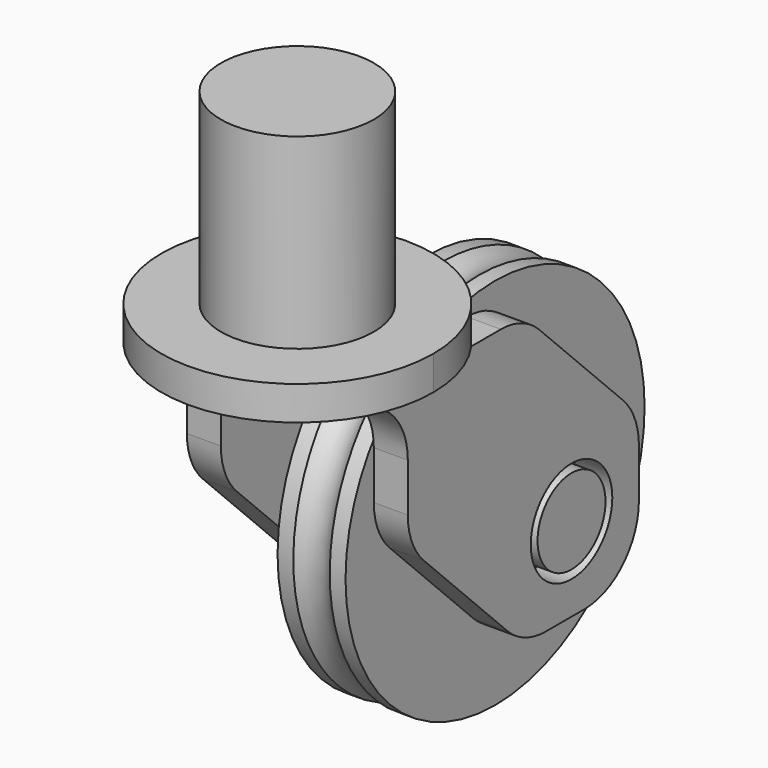
from build123d import *

# Parameters (mm, degrees)
F1_DEPTH  = 13
F2_DEPTH  = 2
F3_DEPTH  = 17
F5_DEPTH  = 14
F6_R      = 4
F7_D      = 6
F8_R      = 11
F8_R_2    = 4.05
F9_DEPTH  = 2
F8_R_3    = 2.5
F10_DEPTH = 6.5
F8_R_4    = 4
F11_DEPTH = 4
F13_R     = 1.5


with BuildPart() as f1:
    # F0 (on Top) → F1 (new body)
    with BuildSketch(Plane.XY):
        with BuildLine():
            ThreePointArc((-4.5, 0), (0, -4.5), (4.5, 0))
            ThreePointArc((4.5, 0), (0, 4.5), (-4.5, 0))
        make_face()
    extrude(amount=F1_DEPTH)

    # F0 (on Top) → F2 (join)
    with BuildSketch(Plane.XY):
        with BuildLine():
            ThreePointArc((-4.5, 0), (0, 4.5), (4.5, 0))
            Line((4.5, 0), (4.5, 6.6143782777))
            ThreePointArc((4.5, 6.6143782777), (0, 8), (-4.5, 6.6143782777))
            Line((-4.5, 6.6143782777), (-4.5, 0))
        make_face()
        with BuildLine():
            Line((-6.5, 0), (-4.5, 0))
            Line((-4.5, 0), (-4.5, 6.6143782777))
            ThreePointArc((-4.5, 6.6143782777), (-5.5858120852, 5.7270152217), (-6.5, 4.6636895265))
            Line((-6.5, 4.6636895265), (-6.5, 0))
        make_face()
        with BuildLine():
            Line((6.5, 0), (4.5, 0))
            ThreePointArc((4.5, 0), (0, -4.5), (-4.5, 0))
            Line((-4.5, 0), (-6.5, 0))
            Line((-6.5, 0), (-6.5, 4.6636895265))
            ThreePointArc((-6.5, 4.6636895265), (-2.4494897428, -7.6157731059), (8, 0))
            ThreePointArc((8, 0), (7.6157731059, 2.4494897428), (6.5, 4.6636895265))
            Line((6.5, 4.6636895265), (6.5, 0))
        make_face()
        with BuildLine():
            Line((4.5, 6.6143782777), (4.5, 0))
            Line((4.5, 0), (6.5, 0))
            Line((6.5, 0), (6.5, 4.6636895265))
            ThreePointArc((6.5, 4.6636895265), (5.5858120852, 5.7270152217), (4.5, 6.6143782777))
        make_face()
    extrude(amount=F2_DEPTH)

    # F0 (on Top) → F3 (join)
    with BuildSketch(Plane.XY):
        with BuildLine():
            ThreePointArc((-6.5, 4.6636895265), (-5.5858120852, 5.7270152217), (-4.5, 6.6143782777))
            Line((-4.5, 6.6143782777), (-4.5, 17))
            Line((-4.5, 17), (-6.5, 17))
            Line((-6.5, 17), (-6.5, 4.6636895265))
        make_face()
        with BuildLine():
            Line((4.5, 17), (4.5, 6.6143782777))
            ThreePointArc((4.5, 6.6143782777), (5.5858120852, 5.7270152217), (6.5, 4.6636895265))
            Line((6.5, 4.6636895265), (6.5, 17))
            Line((6.5, 17), (4.5, 17))
        make_face()
        with BuildLine():
            Line((-6.5, 0), (-4.5, 0))
            Line((-4.5, 0), (-4.5, 6.6143782777))
            ThreePointArc((-4.5, 6.6143782777), (-5.5858120852, 5.7270152217), (-6.5, 4.6636895265))
            Line((-6.5, 4.6636895265), (-6.5, 0))
        make_face()
        with BuildLine():
            Line((4.5, 6.6143782777), (4.5, 0))
            Line((4.5, 0), (6.5, 0))
            Line((6.5, 0), (6.5, 4.6636895265))
            ThreePointArc((6.5, 4.6636895265), (5.5858120852, 5.7270152217), (4.5, 6.6143782777))
        make_face()
    extrude(amount=-F3_DEPTH)

    # F4 (on face) → F5 (cut)
    with BuildSketch(Plane(origin=(-6.5, 0, 0), x_dir=(0, -1, 0), z_dir=(-1, 0, 0))):
        Polygon((-17, 0), (-17, -8.5), (-8.5, 0), align=None)
        Polygon((0, -17), (0, -8.5), (-8.5, -17), align=None)
    extrude(amount=-F5_DEPTH, mode=Mode.SUBTRACT)

    # F6
    f6_edges = [f1.edges().sort_by_distance(p)[0] for p in [
        (-5.5, 17, -17),
        (5.5, 17, -17),
        (-5.5, 0, 0),
        (5.5, 0, 0),
        (-5.5, 0, -8.5),
        (5.5, 0, -8.5),
        (5.5, 8.5, -17),
        (-5.5, 8.5, -17),
        (5.5, 17, -8.5),
        (-5.5, 17, -8.5),
        (5.5, 8.5, 0),
        (-5.5, 8.5, 0),
    ]]
    fillet(f6_edges, radius=F6_R)

    # F7 (through all)
    with Locations(Plane(origin=(-6.5, 0, 0), x_dir=(0, -1, 0), z_dir=(-1, 0, 0))):
        with Locations((-12.0428986898, -12.0576173155)):
            Hole(F7_D / 2)


with BuildPart() as f9:
    # F8 (on Right) → F9 (new body, symmetric)
    with BuildSketch(Plane.YZ):
        with Locations((12.0428986898, -12.0576173155)):
            Circle(F8_R)
        with Locations((12.0428986898, -12.0576173155)):
            Circle(F8_R_2, mode=Mode.SUBTRACT)
    extrude(amount=F9_DEPTH, both=True)

    # F13 (on offset) → F14 (revolve, cut)
    with BuildSketch(Plane.XZ.offset(-11)):
        with Locations((0, -24.0576173155)):
            Circle(F13_R)
    revolve(axis=Axis((2, 12.0428986898, -12.0576173155), (1, 0, 0)), mode=Mode.SUBTRACT)


with BuildPart() as f10:
    # F8 (on Right) → F10 (new body, symmetric)
    with BuildSketch(Plane.YZ):
        with Locations((12.0428986898, -12.0576173155)):
            Circle(F8_R_3)
    extrude(amount=F10_DEPTH, both=True)

    # F8 (on Right) → F11 (join, symmetric)
    with BuildSketch(Plane.YZ):
        with Locations((12.0428986898, -12.0576173155)):
            Circle(F8_R_4)
        with Locations((12.0428986898, -12.0576173155)):
            Circle(F8_R_3, mode=Mode.SUBTRACT)
    extrude(amount=F11_DEPTH, both=True)


solid = Compound([f1.part, f9.part, f10.part])
